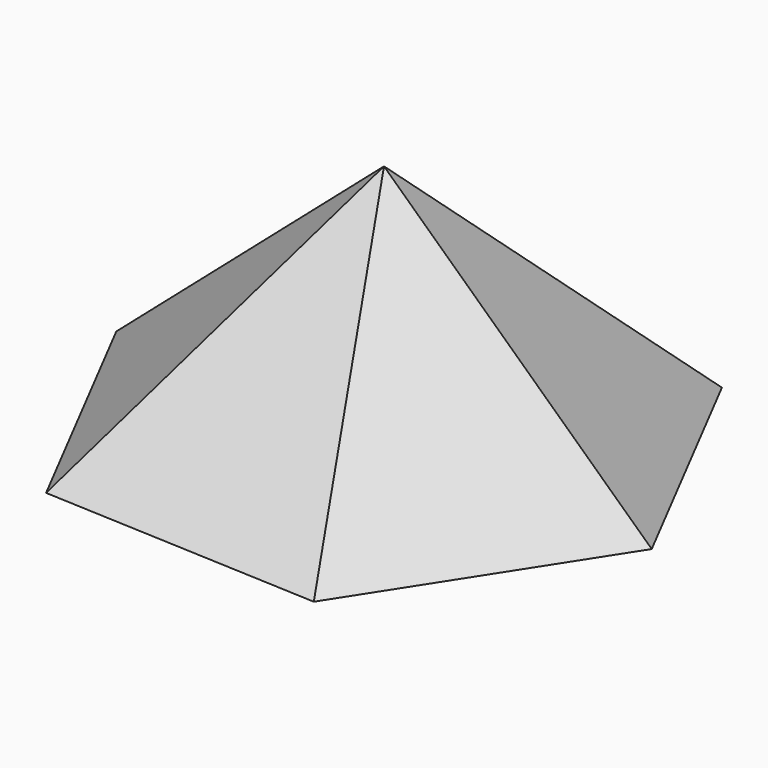
from build123d import *


with BuildPart() as f3:
    # F0 (on Top) → F3 section 0
    with BuildSketch(Plane.XY, mode=Mode.PRIVATE) as f3_s0:
        Polygon((-5.2974935645, 10.2601118545), (-11.5342642939, 0.542291924), (-6.2367707294, -9.7178199305), (5.2974935645, -10.2601118545), (11.5342642939, -0.542291924), (6.2367707294, 9.7178199305), align=None)
    loft([f3_s0.sketch, Vertex(0, 0, 10)])


solid = f3.part
